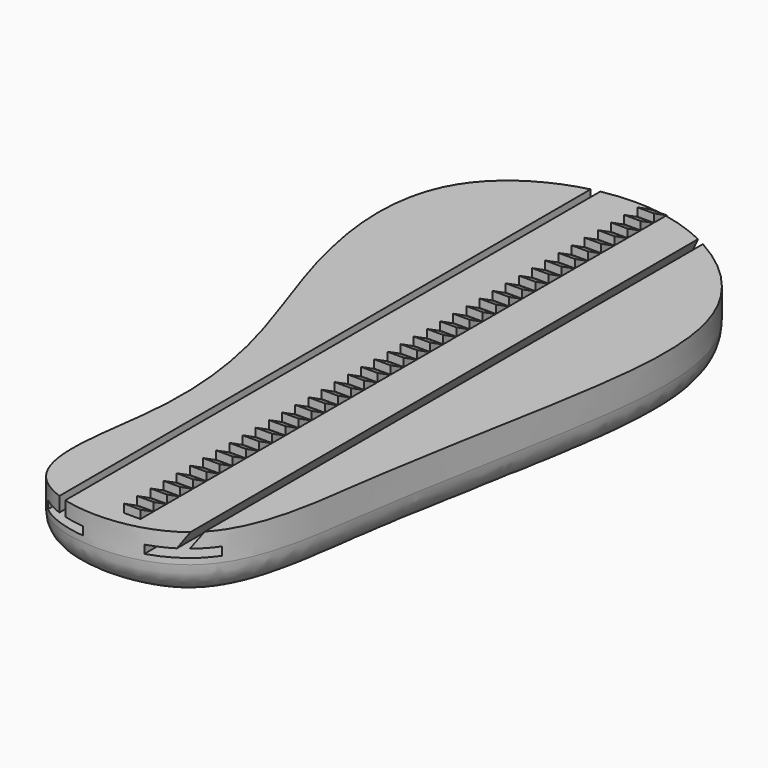
from build123d import *

# Parameters (mm, degrees)
F1_DEPTH      = 9.525
F2_R          = 5.08
F4_DEPTH      = 41.833616476
F4_DEPTH_BACK = 62.5722982436
F7_DEPTH      = 1.27


with BuildPart() as f1:
    # F0 (on Top) → F1 (new body)
    with BuildSketch(Plane.XY):
        with BuildLine():
            add(Edge.make_bspline(
                [(-19.8181457818, 9.1255642474), (-21.6913101918, 17.0916254039), (-23.0280629834, 34.7166818452), (3.9061106439, 46.5389371645), (30.6003252356, 29.2718518116), (27.9148447601, -0.9751801152), (20.959476839, -32.8334090124), (18.3933363928, -64.1805111199), (-15.8935665859, -63.1670764663), (-8.4172546193, -35.956260573), (-11.6136464891, -13.4979246387), (-17.9099211209, 1.0104013353), (-19.8181457818, 9.1255642474)],
                knots=[0, 0, 0, 0, 0.0957385417, 0.192533473, 0.2949798395, 0.3996910778, 0.5173643175, 0.620670135, 0.7128308823, 0.8058151275, 0.9024695081, 1, 1, 1, 1], degree=3))
        make_face()
    extrude(amount=F1_DEPTH)

    # F2
    f2_edges = [f1.edges().sort_by_distance(p)[0] for p in [
        (22.930374, -25.336977, 0),
    ]]
    fillet(f2_edges, radius=F2_R)

    # F3 (on Front) → F4 (cut, two sides)
    with BuildSketch(Plane.XZ) as f4_sk:
        Polygon((-8.2057012741, 7.2674243711), (-8.2057012741, 5.9974243711), (-0.5857012741, 5.9974243711), (-0.5857012741, 7.2674243711), (-3.7861012741, 7.2674243711), (-3.7861012741, 13.8412946235), (-5.0561012741, 13.8412946235), (-5.0561012741, 7.2674243711), align=None)
        Polygon((11.8464205279, 7.2674243711), (8.1585189328, 7.2674243711), (8.1585189328, 5.9974243711), (15.7785201703, 5.9974243711), (15.7785201703, 7.2674243711), (13.1164205279, 7.2674243711), (17.0010384482, 13.8412946235), (15.7310384482, 13.8412946235), align=None)
    extrude(amount=-F4_DEPTH, mode=Mode.SUBTRACT)
    extrude(f4_sk.sketch, amount=F4_DEPTH_BACK, mode=Mode.SUBTRACT)

    # F6 (on offset) → F7 (join, symmetric)
    with BuildSketch(Plane.YZ.offset(5.08)):
        Polygon((41.5405707741, 8.5993949324), (41.5405707741, 9.4965914902), (39.0005707741, 10.795), (39.0005707741, 9.525), (39.0002332586, 9.4967640229), (39.0005707741, 9.4965914902), (39.0005707741, 8.5993949324), align=None)
        Polygon((38.9895066619, 8.5993949324), (39.0005707741, 8.5993949324), (39.0005707741, 9.4965914902), (39.0002332586, 9.4967640229), align=None)
        Polygon((38.9895066619, 8.5993949324), (39.0002332586, 9.4967640229), (36.4605707741, 10.795), (36.4605707741, 9.525), (36.4602332586, 9.4967640229), (36.4605707741, 9.4965914902), (36.4605707741, 8.5993949324), align=None)
        Polygon((36.4495066619, 8.5993949324), (36.4605707741, 8.5993949324), (36.4605707741, 9.4965914902), (36.4602332586, 9.4967640229), align=None)
        Polygon((33.9205707741, 8.5993949324), (36.4495066619, 8.5993949324), (36.4602332586, 9.4967640229), (33.9205707741, 10.795), (33.9205707741, 9.525), (33.9202332586, 9.4967640229), (33.9205707741, 9.4965914902), align=None)
        Polygon((33.9095066619, 8.5993949324), (33.9205707741, 8.5993949324), (33.9205707741, 9.4965914902), (33.9202332586, 9.4967640229), align=None)
        Polygon((31.3805707741, 8.5993949324), (33.9095066619, 8.5993949324), (33.9202332586, 9.4967640229), (31.3805707741, 10.795), (31.3805707741, 9.525), (31.3802332586, 9.4967640229), (31.3805707741, 9.4965914902), align=None)
        Polygon((31.3695066619, 8.5993949324), (31.3805707741, 8.5993949324), (31.3805707741, 9.4965914902), (31.3802332586, 9.4967640229), align=None)
        Polygon((28.8405707741, 8.5993949324), (31.3695066619, 8.5993949324), (31.3802332586, 9.4967640229), (28.8405707741, 10.795), (28.8405707741, 9.525), (28.8402332586, 9.4967640229), (28.8405707741, 9.4965914902), align=None)
        Polygon((28.8295066619, 8.5993949324), (28.8405707741, 8.5993949324), (28.8405707741, 9.4965914902), (28.8402332586, 9.4967640229), align=None)
        Polygon((26.3005707741, 8.5993949324), (28.8295066619, 8.5993949324), (28.8402332586, 9.4967640229), (26.3005707741, 10.795), (26.3005707741, 9.525), (26.3002332586, 9.4967640229), (26.3005707741, 9.4965914902), align=None)
        Polygon((26.2895066619, 8.5993949324), (26.3005707741, 8.5993949324), (26.3005707741, 9.4965914902), (26.3002332586, 9.4967640229), align=None)
        Polygon((23.7605707741, 8.5993949324), (26.2895066619, 8.5993949324), (26.3002332586, 9.4967640229), (23.7605707741, 10.795), (23.7605707741, 9.525), (23.7602332586, 9.4967640229), (23.7605707741, 9.4965914902), align=None)
        Polygon((23.7495066619, 8.5993949324), (23.7605707741, 8.5993949324), (23.7605707741, 9.4965914902), (23.7602332586, 9.4967640229), align=None)
        Polygon((21.2205707741, 8.5993949324), (23.7495066619, 8.5993949324), (23.7602332586, 9.4967640229), (21.2205707741, 10.795), (21.2205707741, 9.525), (21.2202332586, 9.4967640229), (21.2205707741, 9.4965914902), align=None)
        Polygon((21.2095066619, 8.5993949324), (21.2205707741, 8.5993949324), (21.2205707741, 9.4965914902), (21.2202332586, 9.4967640229), align=None)
        Polygon((18.6805707741, 8.5993949324), (21.2095066619, 8.5993949324), (21.2202332586, 9.4967640229), (18.6805707741, 10.795), (18.6805707741, 9.525), (18.6802332586, 9.4967640229), (18.6805707741, 9.4965914902), align=None)
        Polygon((18.6695066619, 8.5993949324), (18.6805707741, 8.5993949324), (18.6805707741, 9.4965914902), (18.6802332586, 9.4967640229), align=None)
        Polygon((16.1405707741, 8.5993949324), (18.6695066619, 8.5993949324), (18.6802332586, 9.4967640229), (16.1405707741, 10.795), (16.1405707741, 9.525), (16.1402332586, 9.4967640229), (16.1405707741, 9.4965914902), align=None)
        Polygon((16.1295066619, 8.5993949324), (16.1405707741, 8.5993949324), (16.1405707741, 9.4965914902), (16.1402332586, 9.4967640229), align=None)
        Polygon((13.6005707741, 8.5993949324), (16.1295066619, 8.5993949324), (16.1402332586, 9.4967640229), (13.6005707741, 10.795), (13.6005707741, 9.525), (13.6002332586, 9.4967640229), (13.6005707741, 9.4965914902), align=None)
        Polygon((13.5895066619, 8.5993949324), (13.6005707741, 8.5993949324), (13.6005707741, 9.4965914902), (13.6002332586, 9.4967640229), align=None)
        Polygon((11.0605707741, 8.5993949324), (13.5895066619, 8.5993949324), (13.6002332586, 9.4967640229), (11.0605707741, 10.795), (11.0605707741, 9.525), (11.0602332586, 9.4967640229), (11.0605707741, 9.4965914902), align=None)
        Polygon((11.0495066619, 8.5993949324), (11.0605707741, 8.5993949324), (11.0605707741, 9.4965914902), (11.0602332586, 9.4967640229), align=None)
        Polygon((8.5205707741, 8.5993949324), (11.0495066619, 8.5993949324), (11.0602332586, 9.4967640229), (8.5205707741, 10.795), (8.5205707741, 9.525), (8.5202332586, 9.4967640229), (8.5205707741, 9.4965914902), align=None)
        Polygon((8.5095066619, 8.5993949324), (8.5205707741, 8.5993949324), (8.5205707741, 9.4965914902), (8.5202332586, 9.4967640229), align=None)
        Polygon((5.9805707741, 8.5993949324), (8.5095066619, 8.5993949324), (8.5202332586, 9.4967640229), (5.9805707741, 10.795), (5.9805707741, 9.525), (5.9802332586, 9.4967640229), (5.9805707741, 9.4965914902), align=None)
        Polygon((5.9695066619, 8.5993949324), (5.9805707741, 8.5993949324), (5.9805707741, 9.4965914902), (5.9802332586, 9.4967640229), align=None)
        Polygon((3.4405707741, 8.5993949324), (5.9695066619, 8.5993949324), (5.9802332586, 9.4967640229), (3.4405707741, 10.795), (3.4405707741, 9.525), (3.4402332586, 9.4967640229), (3.4405707741, 9.4965914902), align=None)
        Polygon((3.4295066619, 8.5993949324), (3.4405707741, 8.5993949324), (3.4405707741, 9.4965914902), (3.4402332586, 9.4967640229), align=None)
        Polygon((0.9005707741, 8.5993949324), (3.4295066619, 8.5993949324), (3.4402332586, 9.4967640229), (0.9005707741, 10.795), (0.9005707741, 9.525), (0.9002332586, 9.4967640229), (0.9005707741, 9.4965914902), align=None)
        Polygon((0.8895066619, 8.5993949324), (0.9005707741, 8.5993949324), (0.9005707741, 9.4965914902), (0.9002332586, 9.4967640229), align=None)
        Polygon((-1.6394292259, 8.5993949324), (0.8895066619, 8.5993949324), (0.9002332586, 9.4967640229), (-1.6394292259, 10.795), (-1.6394292259, 9.525), (-1.6397667414, 9.4967640229), (-1.6394292259, 9.4965914902), align=None)
        Polygon((-1.6504933381, 8.5993949324), (-1.6394292259, 8.5993949324), (-1.6394292259, 9.4965914902), (-1.6397667414, 9.4967640229), align=None)
        Polygon((-4.1794292259, 8.5993949324), (-1.6504933381, 8.5993949324), (-1.6397667414, 9.4967640229), (-4.1794292259, 10.795), (-4.1794292259, 9.525), (-4.1797667414, 9.4967640229), (-4.1794292259, 9.4965914902), align=None)
        Polygon((-4.1904933381, 8.5993949324), (-4.1794292259, 8.5993949324), (-4.1794292259, 9.4965914902), (-4.1797667414, 9.4967640229), align=None)
        Polygon((-6.7194292259, 8.5993949324), (-4.1904933381, 8.5993949324), (-4.1797667414, 9.4967640229), (-6.7194292259, 10.795), (-6.7194292259, 9.525), (-6.7197667414, 9.4967640229), (-6.7194292259, 9.4965914902), align=None)
        Polygon((-6.7304933381, 8.5993949324), (-6.7194292259, 8.5993949324), (-6.7194292259, 9.4965914902), (-6.7197667414, 9.4967640229), align=None)
        Polygon((-9.2594292259, 8.5993949324), (-6.7304933381, 8.5993949324), (-6.7197667414, 9.4967640229), (-9.2594292259, 10.795), (-9.2594292259, 9.525), (-9.2597667414, 9.4967640229), (-9.2594292259, 9.4965914902), align=None)
        Polygon((-9.2704933381, 8.5993949324), (-9.2594292259, 8.5993949324), (-9.2594292259, 9.4965914902), (-9.2597667414, 9.4967640229), align=None)
        Polygon((-11.7994292259, 8.5993949324), (-9.2704933381, 8.5993949324), (-9.2597667414, 9.4967640229), (-11.7994292259, 10.795), (-11.7994292259, 9.525), (-11.7997667414, 9.4967640229), (-11.7994292259, 9.4965914902), align=None)
        Polygon((-11.8104933381, 8.5993949324), (-11.7994292259, 8.5993949324), (-11.7994292259, 9.4965914902), (-11.7997667414, 9.4967640229), align=None)
        Polygon((-14.3394292259, 8.5993949324), (-11.8104933381, 8.5993949324), (-11.7997667414, 9.4967640229), (-14.3394292259, 10.795), (-14.3394292259, 9.525), (-14.3397667414, 9.4967640229), (-14.3394292259, 9.4965914902), align=None)
        Polygon((-14.3504933381, 8.5993949324), (-14.3394292259, 8.5993949324), (-14.3394292259, 9.4965914902), (-14.3397667414, 9.4967640229), align=None)
        Polygon((-16.8794292259, 8.5993949324), (-14.3504933381, 8.5993949324), (-14.3397667414, 9.4967640229), (-16.8794292259, 10.795), (-16.8794292259, 9.525), (-16.8797667414, 9.4967640229), (-16.8794292259, 9.4965914902), align=None)
        Polygon((-16.8904933381, 8.5993949324), (-16.8794292259, 8.5993949324), (-16.8794292259, 9.4965914902), (-16.8797667414, 9.4967640229), align=None)
        Polygon((-19.4194292259, 8.5993949324), (-16.8904933381, 8.5993949324), (-16.8797667414, 9.4967640229), (-19.4194292259, 10.795), (-19.4194292259, 9.525), (-19.4197667414, 9.4967640229), (-19.4194292259, 9.4965914902), align=None)
        Polygon((-19.4304933381, 8.5993949324), (-19.4194292259, 8.5993949324), (-19.4194292259, 9.4965914902), (-19.4197667414, 9.4967640229), align=None)
        Polygon((-21.9594292259, 8.5993949324), (-19.4304933381, 8.5993949324), (-19.4197667414, 9.4967640229), (-21.9594292259, 10.795), (-21.9594292259, 9.525), (-21.9597667414, 9.4967640229), (-21.9594292259, 9.4965914902), align=None)
        Polygon((-21.9704933381, 8.5993949324), (-21.9594292259, 8.5993949324), (-21.9594292259, 9.4965914902), (-21.9597667414, 9.4967640229), align=None)
        Polygon((-24.4994292259, 8.5993949324), (-21.9704933381, 8.5993949324), (-21.9597667414, 9.4967640229), (-24.4994292259, 10.795), (-24.4994292259, 9.525), (-24.4997667414, 9.4967640229), (-24.4994292259, 9.4965914902), align=None)
        Polygon((-24.5104933381, 8.5993949324), (-24.4994292259, 8.5993949324), (-24.4994292259, 9.4965914902), (-24.4997667414, 9.4967640229), align=None)
        Polygon((-27.0394292259, 8.5993949324), (-24.5104933381, 8.5993949324), (-24.4997667414, 9.4967640229), (-27.0394292259, 10.795), (-27.0394292259, 9.525), (-27.0397667414, 9.4967640229), (-27.0394292259, 9.4965914902), align=None)
        Polygon((-27.0504933381, 8.5993949324), (-27.0394292259, 8.5993949324), (-27.0394292259, 9.4965914902), (-27.0397667414, 9.4967640229), align=None)
        Polygon((-29.5794292259, 8.5993949324), (-27.0504933381, 8.5993949324), (-27.0397667414, 9.4967640229), (-29.5794292259, 10.795), (-29.5794292259, 9.525), (-29.5797667414, 9.4967640229), (-29.5794292259, 9.4965914902), align=None)
        Polygon((-29.5904933381, 8.5993949324), (-29.5794292259, 8.5993949324), (-29.5794292259, 9.4965914902), (-29.5797667414, 9.4967640229), align=None)
        Polygon((-32.1194292259, 8.5993949324), (-29.5904933381, 8.5993949324), (-29.5797667414, 9.4967640229), (-32.1194292259, 10.795), (-32.1194292259, 9.525), (-32.1197667414, 9.4967640229), (-32.1194292259, 9.4965914902), align=None)
        Polygon((-32.1304933381, 8.5993949324), (-32.1194292259, 8.5993949324), (-32.1194292259, 9.4965914902), (-32.1197667414, 9.4967640229), align=None)
        Polygon((-34.6594292259, 8.5993949324), (-32.1304933381, 8.5993949324), (-32.1197667414, 9.4967640229), (-34.6594292259, 10.795), (-34.6594292259, 9.525), (-34.6597667414, 9.4967640229), (-34.6594292259, 9.4965914902), align=None)
        Polygon((-34.6704933381, 8.5993949324), (-34.6594292259, 8.5993949324), (-34.6594292259, 9.4965914902), (-34.6597667414, 9.4967640229), align=None)
        Polygon((-37.1994292259, 8.5993949324), (-34.6704933381, 8.5993949324), (-34.6597667414, 9.4967640229), (-37.1994292259, 10.795), (-37.1994292259, 9.525), (-37.1997667414, 9.4967640229), (-37.1994292259, 9.4965914902), align=None)
        Polygon((-37.2104933381, 8.5993949324), (-37.1994292259, 8.5993949324), (-37.1994292259, 9.4965914902), (-37.1997667414, 9.4967640229), align=None)
        Polygon((-39.7394292259, 8.5993949324), (-37.2104933381, 8.5993949324), (-37.1997667414, 9.4967640229), (-39.7394292259, 10.795), (-39.7394292259, 9.525), (-39.7397667414, 9.4967640229), (-39.7394292259, 9.4965914902), align=None)
        Polygon((-39.7504933381, 8.5993949324), (-39.7394292259, 8.5993949324), (-39.7394292259, 9.4965914902), (-39.7397667414, 9.4967640229), align=None)
        Polygon((-42.2794292259, 8.5993949324), (-39.7504933381, 8.5993949324), (-39.7397667414, 9.4967640229), (-42.2794292259, 10.795), (-42.2794292259, 9.525), (-42.2797667414, 9.4967640229), (-42.2794292259, 9.4965914902), align=None)
        Polygon((-42.2904933381, 8.5993949324), (-42.2794292259, 8.5993949324), (-42.2794292259, 9.4965914902), (-42.2797667414, 9.4967640229), align=None)
        Polygon((-44.8194292259, 8.5993949324), (-42.2904933381, 8.5993949324), (-42.2797667414, 9.4967640229), (-44.8194292259, 10.795), (-44.8194292259, 9.525), (-44.8197667414, 9.4967640229), (-44.8194292259, 9.4965914902), align=None)
        Polygon((-44.8304933381, 8.5993949324), (-44.8194292259, 8.5993949324), (-44.8194292259, 9.4965914902), (-44.8197667414, 9.4967640229), align=None)
        Polygon((-47.3594292259, 8.5993949324), (-44.8304933381, 8.5993949324), (-44.8197667414, 9.4967640229), (-47.3594292259, 10.795), (-47.3594292259, 9.525), (-47.3597667414, 9.4967640229), (-47.3594292259, 9.4965914902), align=None)
        Polygon((-47.3704933381, 8.5993949324), (-47.3594292259, 8.5993949324), (-47.3594292259, 9.4965914902), (-47.3597667414, 9.4967640229), align=None)
        Polygon((-49.8994292259, 8.5993949324), (-47.3704933381, 8.5993949324), (-47.3597667414, 9.4967640229), (-49.8994292259, 10.795), (-49.8994292259, 9.525), (-49.8997667414, 9.4967640229), (-49.8994292259, 9.4965914902), align=None)
        Polygon((-49.9104933381, 8.5993949324), (-49.8994292259, 8.5993949324), (-49.8994292259, 9.4965914902), (-49.8997667414, 9.4967640229), align=None)
        Polygon((-52.4394292259, 8.5993949324), (-49.9104933381, 8.5993949324), (-49.8997667414, 9.4967640229), (-52.4394292259, 10.795), (-52.4394292259, 9.525), (-52.4397667414, 9.4967640229), (-52.4394292259, 9.4965914902), align=None)
        Polygon((-52.4504933381, 8.5993949324), (-52.4394292259, 8.5993949324), (-52.4394292259, 9.4965914902), (-52.4397667414, 9.4967640229), align=None)
        Polygon((-54.9794292259, 8.5993949324), (-52.4504933381, 8.5993949324), (-52.4397667414, 9.4967640229), (-54.9794292259, 10.795), (-54.9794292259, 9.525), (-54.9797667414, 9.4967640229), (-54.9794292259, 9.4965914902), align=None)
        Polygon((-54.9904933381, 8.5993949324), (-54.9794292259, 8.5993949324), (-54.9794292259, 9.4965914902), (-54.9797667414, 9.4967640229), align=None)
        Polygon((-57.5194292259, 8.5993949324), (-54.9904933381, 8.5993949324), (-54.9797667414, 9.4967640229), (-57.5194292259, 10.795), (-57.5194292259, 9.525), (-57.5197667414, 9.4967640229), (-57.5194292259, 9.4965914902), align=None)
        Polygon((-57.5304933381, 8.5993949324), (-57.5194292259, 8.5993949324), (-57.5194292259, 9.4965914902), (-57.5197667414, 9.4967640229), align=None)
        Polygon((-60.0704933381, 8.5993949324), (-57.5304933381, 8.5993949324), (-57.5197667414, 9.4967640229), (-60.0594292259, 10.795), (-60.0594292259, 9.525), align=None)
    extrude(amount=F7_DEPTH, both=True)


solid = f1.part
